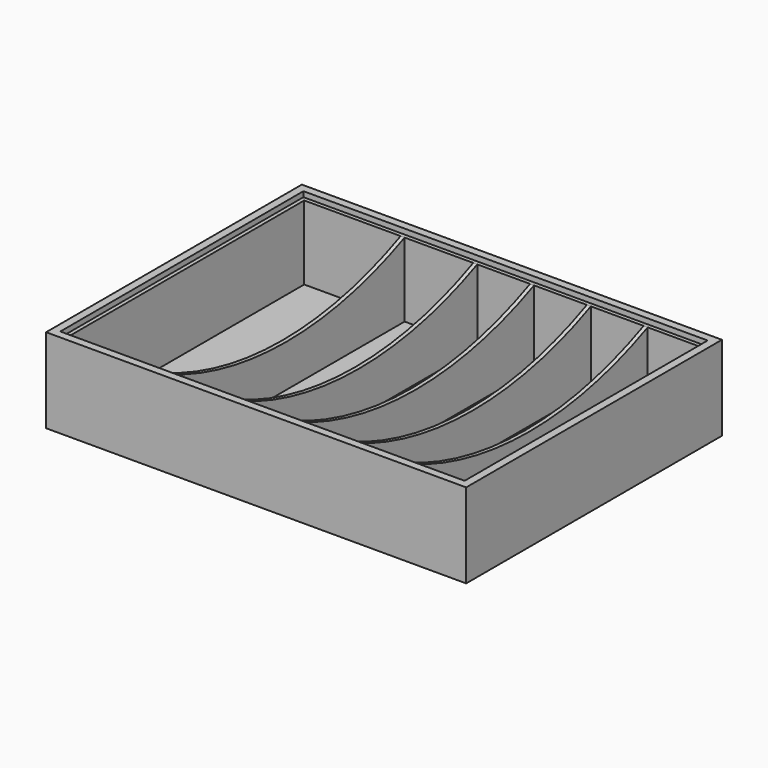
from build123d import *

# Parameters (mm, degrees)
F0_W     = 504.825
F0_H     = 384.175
F0_W_2   = 485.775
F0_H_2   = 365.125
F1_DEPTH = 95.25
F0_W_3   = 115.8875
F0_H_3   = 355.6
F0_W_4   = 82.55
F0_W_5   = 63.5
F2_DEPTH = 88.9
F3_W     = 504.825
F3_H     = 384.175
F4_DEPTH = 6.35
F6_DEPTH = 296.8625


with BuildPart() as f1:
    # F0 (on Top) → F1 (new body)
    with BuildSketch(Plane.XY):
        with Locations((108.3223706484, 74.7603473186)):
            Rectangle(F0_W, F0_H)
        with Locations((108.3223706484, 74.7603473186)):
            Rectangle(F0_W_2, F0_H_2, mode=Mode.SUBTRACT)
    extrude(amount=F1_DEPTH)

    # F3 (on face) → F4 (join)
    with BuildSketch(Plane.XY):
        with Locations((108.3223706484, 74.7603473186)):
            Rectangle(F3_W, F3_H)
    extrude(amount=-F4_DEPTH)


with BuildPart() as f2:
    # F0 (on Top) → F2 (new body)
    with BuildSketch(Plane.XY):
        with Locations((108.3223706484, 74.7603473186)):
            Rectangle(F0_W_2, F0_H_2)
        with Locations((-71.8588793516, 74.7603473186)):
            Rectangle(F0_W_3, F0_H_3, mode=Mode.SUBTRACT)
        with Locations((32.1223706484, 74.7603473186)):
            Rectangle(F0_W_4, F0_H_3, mode=Mode.SUBTRACT)
        with Locations((109.9098706484, 74.7603473186)):
            Rectangle(F0_W_5, F0_H_3, mode=Mode.SUBTRACT)
        with Locations((178.1723706484, 74.7603473186)):
            Rectangle(F0_W_5, F0_H_3, mode=Mode.SUBTRACT)
        with Locations((246.4348706484, 74.7603473186)):
            Rectangle(F0_W_5, F0_H_3, mode=Mode.SUBTRACT)
        with Locations((314.6973706484, 74.7603473186)):
            Rectangle(F0_W_5, F0_H_3, mode=Mode.SUBTRACT)
    extrude(amount=F2_DEPTH)

    # F5 (on face) → F6 (cut, through all)
    with BuildSketch(Plane.YZ.offset(282.9473706484)):
        with BuildLine():
            Line((252.5603473186, 88.9), (-103.0396526814, 88.9))
            ThreePointArc((-103.0396526814, 88.9), (74.7603473186, 50.8), (252.5603473186, 88.9))
        make_face()
    extrude(amount=-F6_DEPTH, mode=Mode.SUBTRACT)


solid = Compound([f1.part, f2.part])
